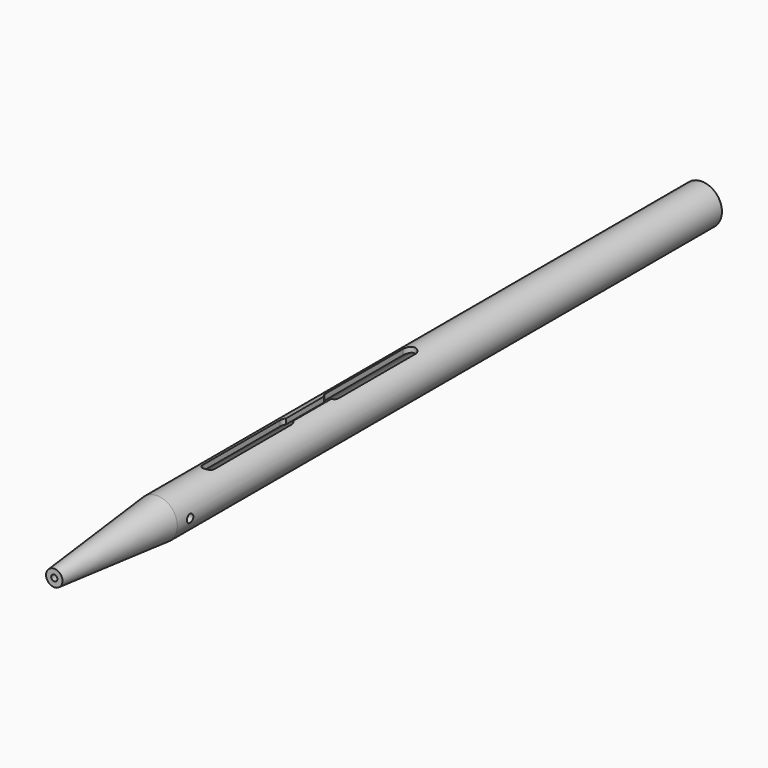
from build123d import *

# Parameters (mm, degrees)
F0_R          = 3.96875
F0_R_2        = 2.95275
F1_DEPTH      = 134.366
F3_DEPTH      = 3.96975
F3_DEPTH_BACK = 3.96975
F7_R          = 0.79375
F8_DEPTH      = 12.7
F9_DEPTH      = 3.9697501215


# Not quite as in the source:
# - the program builds the solid bodies; features that only make, move or delete a surface that nothing else refers to are left out


with BuildPart() as f1:
    # F0 (on Front) → F1 (new body)
    with BuildSketch(Plane.XZ):
        Circle(F0_R)
        Circle(F0_R_2, mode=Mode.SUBTRACT)
    extrude(amount=-F1_DEPTH)

    # F2 (on Top) → F3 (cut, two sides)
    with BuildSketch(Plane.XY) as f3_sk:
        with BuildLine():
            ThreePointArc((1.143, 31.75), (0, 32.893), (-1.143, 31.75))
            Line((-1.143, 31.75), (-1.143, 12.7))
            ThreePointArc((-1.143, 12.7), (0, 11.557), (1.143, 12.7))
            Line((1.143, 12.7), (1.143, 31.75))
        make_face()
    extrude(amount=F3_DEPTH, mode=Mode.SUBTRACT)
    extrude(f3_sk.sketch, amount=-F3_DEPTH_BACK, mode=Mode.SUBTRACT)

    # F5 (on Right) → F6 (revolve)
    with BuildSketch(Plane.YZ):
        Polygon((0, 3.96875), (-25.4, 1.6208575107), (-25.4, 0.6048575107), (0, 2.95275), align=None)
    revolve(axis=Axis((0, -12.7, 0), (0, 1, 0)))

    # F7 (on Right) → F8 (cut, symmetric)
    with BuildSketch(Plane.YZ):
        with Locations((3.175, 0)):
            Circle(F7_R)
    extrude(amount=F8_DEPTH, both=True, mode=Mode.SUBTRACT)

    # F4 (on Top) → F9 (cut, through all)
    with BuildSketch(Plane.XY):
        with BuildLine():
            ThreePointArc((1.27, 62.165913868), (0, 63.435913868), (-1.27, 62.165913868))
            Line((-1.27, 62.165913868), (-1.27, 43.115913868))
            ThreePointArc((-1.27, 43.115913868), (-1.1164401975, 42.5105534089), (-0.6928956136, 42.0515851271))
            Line((-0.6928956136, 42.0515851271), (-0.6928956136, 31.9918245077))
            Line((-0.6928956136, 31.9918245077), (0.6928956136, 31.9918245077))
            Line((0.6928956136, 31.9918245077), (0.6928956136, 42.0515851271))
            ThreePointArc((0.6928956136, 42.0515851271), (1.1164401975, 42.5105534089), (1.27, 43.115913868))
            Line((1.27, 43.115913868), (1.27, 62.165913868))
        make_face()
    extrude(amount=F9_DEPTH, mode=Mode.SUBTRACT)


solid = f1.part
